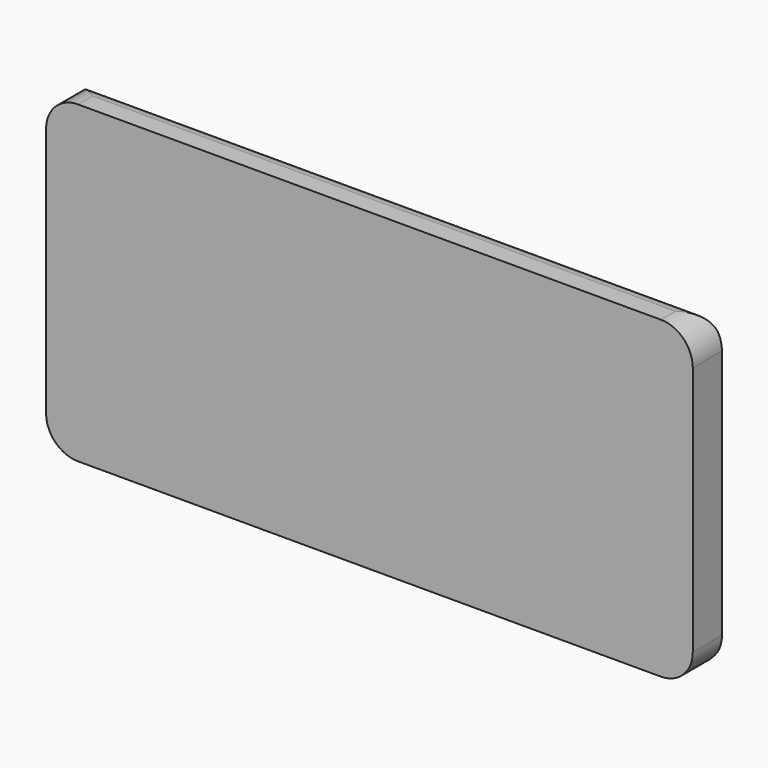
from build123d import *

# Parameters (mm, degrees)
F1_DEPTH      = 4
F1_DEPTH_BACK = 4
F2_T1_DEPTH   = 148


# Not quite as in the source:
# - a fillet or chamfer that OpenCascade refuses, or shapes differently, is made with other operations: its cross-section is extruded or revolved along the edge and cut away or added


with BuildPart() as f1:
    # F0 (on Front) → F1 (new body, two sides)
    with BuildSketch(Plane.XZ) as f1_sk:
        with BuildLine():
            Line((-64, -34.5), (64, -34.5))
            ThreePointArc((64, -34.5), (68.9497474683, -32.4497474683), (71, -27.5))
            Line((71, -27.5), (71, 27.5))
            ThreePointArc((71, 27.5), (68.9497474683, 32.4497474683), (64, 34.5))
            Line((64, 34.5), (-64, 34.5))
            ThreePointArc((-64, 34.5), (-68.9497474683, 32.4497474683), (-71, 27.5))
            Line((-71, 27.5), (-71, -27.5))
            ThreePointArc((-71, -27.5), (-68.9497474683, -32.4497474683), (-64, -34.5))
        make_face()
    extrude(amount=F1_DEPTH)
    extrude(f1_sk.sketch, amount=-F1_DEPTH_BACK)

    # F2: fillet of radius 4 on 2 edges, made by hand

    # F2_s2 → F2_t1 (cut)
    with BuildSketch(Plane.YZ.offset(-74)):
        with BuildLine():
            ThreePointArc((4, 30.5), (2.8284271247, 33.3284271247), (0, 34.5))
            Line((0, 34.5), (4, 34.5))
            Line((4, 34.5), (4, 30.5))
        make_face()
        with BuildLine():
            ThreePointArc((0, -34.5), (2.8284271247, -33.3284271247), (4, -30.5))
            Line((4, -30.5), (4, -34.5))
            Line((4, -34.5), (0, -34.5))
        make_face()
    extrude(amount=F2_T1_DEPTH, mode=Mode.SUBTRACT)


solid = f1.part
